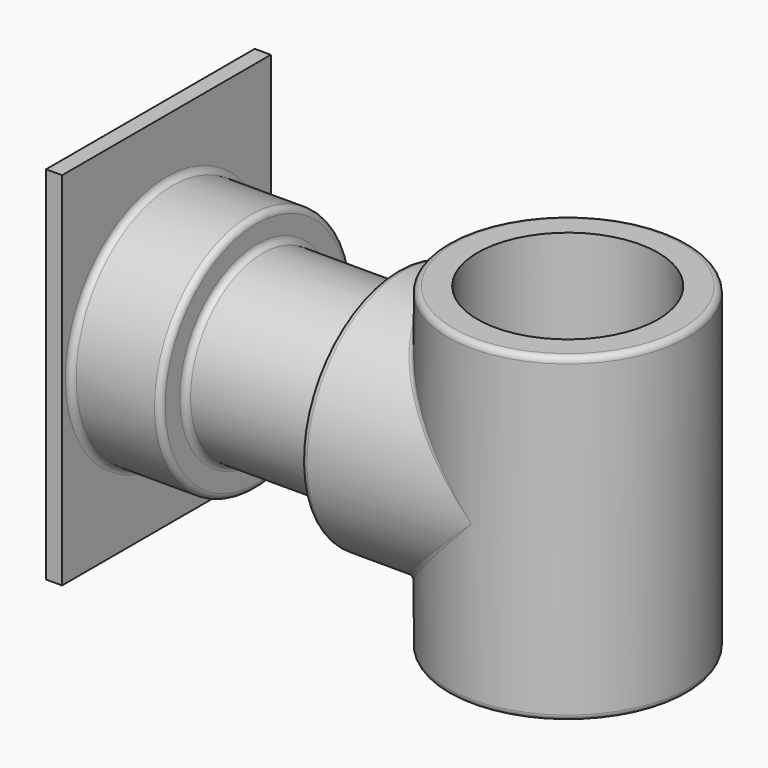
from build123d import *

# Parameters (mm, degrees)
F4_W     = 52
F4_H     = 72
F5_DEPTH = 3.2
F6_F1_R  = 1.2
F6_F2_R  = 1.2
F6_F3_R  = 1.2
F6_F4_R  = 1.2
F6_F5_R  = 1.2
F7_R     = 18
F8_DEPTH = 68.001


with BuildPart() as f1:
    # F0 (on Front) → F1 (revolve)
    with BuildSketch(Plane.XZ):
        with BuildLine():
            Line((-63.2, 24), (-80, 24))
            Line((-80, 24), (-80, 0))
            Line((-80, 0), (0, 0))
            Line((0, 0), (0, 24))
            Line((0, 24), (-32.8, 24))
            ThreePointArc((-32.8, 24), (-33.6485281374, 23.6485281374), (-34, 22.8))
            Line((-34, 22.8), (-34, 18))
            Line((-34, 18), (-62, 18))
            Line((-62, 18), (-62, 22.8))
            ThreePointArc((-62, 22.8), (-62.3514718626, 23.6485281374), (-63.2, 24))
        make_face()
    revolve(axis=Axis((-40, 0, 0), (1, 0, 0)))

    # F2 (on Front) → F3 (revolve)
    with BuildSketch(Plane.XZ):
        with BuildLine():
            Line((0, 32), (-22.8, 32))
            ThreePointArc((-22.8, 32), (-23.6485281374, 31.6485281374), (-24, 30.8))
            Line((-24, 30.8), (-24, -30.8))
            ThreePointArc((-24, -30.8), (-23.6485281374, -31.6485281374), (-22.8, -32))
            Line((-22.8, -32), (0, -32))
            Line((0, -32), (0, 32))
        make_face()
    revolve(axis=Axis((0, 0, 0), (0, 0, -1)))

    # F4 (on face) → F5 (join)
    with BuildSketch(Plane(origin=(-80, 0, 0), x_dir=(0, -1, 0), z_dir=(-1, 0, 0))):
        Rectangle(F4_W, F4_H)
    extrude(amount=F5_DEPTH)

    # F6: fillet of radius 1.2 on 7 edges, made by hand

    # F6_f1
    f6_f1_edges = [f1.edges().sort_by_distance(p)[0] for p in [
        (-80, 0, -24),
    ]]
    fillet(f6_f1_edges, radius=F6_F1_R)

    # F6_f2
    f6_f2_edges = [f1.edges().sort_by_distance(p)[0] for p in [
        (-62, 0, -18),
    ]]
    fillet(f6_f2_edges, radius=F6_F2_R)

    # F6_f3
    f6_f3_edges = [f1.edges().sort_by_distance(p)[0] for p in [
        (-34, 0, -18),
    ]]
    fillet(f6_f3_edges, radius=F6_F3_R)

    # F6_f4
    f6_f4_edges = [f1.edges().sort_by_distance(p)[0] for p in [
        (-16.9705627499, -16.9705627471, 16.9705627499),
        (-16.9705627485, 16.9705627485, 16.9705627485),
    ]]
    fillet(f6_f4_edges, radius=F6_F4_R)

    # F6_f5
    f6_f5_edges = [f1.edges().sort_by_distance(p)[0] for p in [
        (-16.9705627499, 16.9705627471, -16.9705627499),
        (-16.9705627485, -16.9705627485, -16.9705627485),
    ]]
    fillet(f6_f5_edges, radius=F6_F5_R)

    # F7 (on face) → F8 (cut, through all)
    with BuildSketch(Plane.XY.offset(32)):
        Circle(F7_R)
    extrude(amount=-F8_DEPTH, mode=Mode.SUBTRACT)


solid = f1.part
